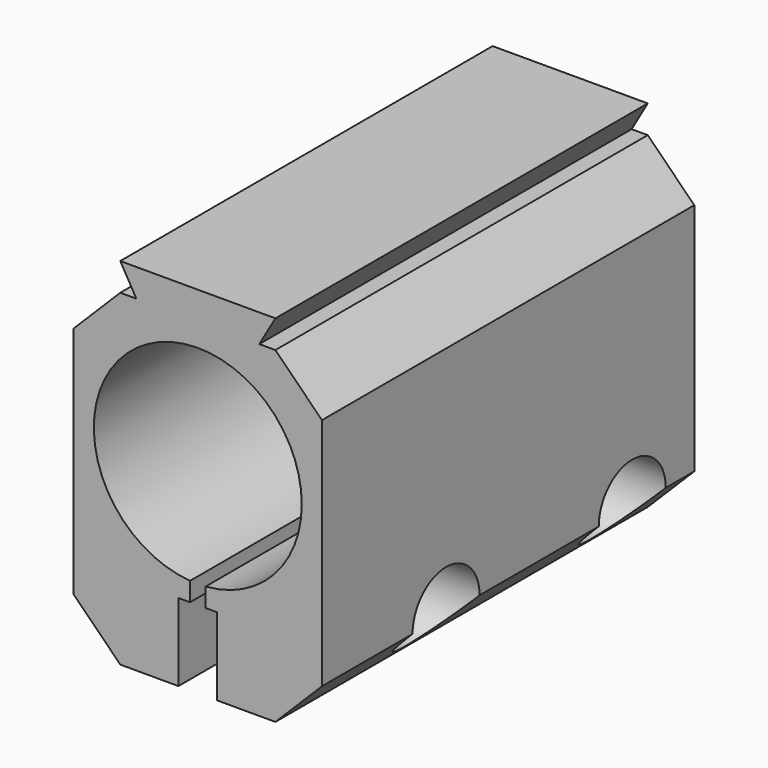
from build123d import *

# Parameters (mm, degrees)
F0_R     = 8.509
F1_DEPTH = 38.1
F3_DEPTH = 6.35
F5_DEPTH = 5.08
F6_DEPTH = 20.321
F8_DEPTH = 8.897727111


# Not quite as in the source:
# - a feature names something its author has since deleted; it is built from what else it names


with BuildPart() as f1:
    # F0 (on Front) → F1 (new body)
    with BuildSketch(Plane.XZ):
        Polygon((5.0301772846, 10.414), (-5.0301772846, 10.414), (-6.35, 10.414), (-10.16, 6.604), (-10.16, -12.5681449387), (-6.3451449387, -16.383), (6.35, -16.383), (10.16, -12.573), (10.16, 6.604), (6.35, 10.414), align=None)
        Circle(F0_R, mode=Mode.SUBTRACT)
        Polygon((6.35, 12.7), (-6.35, 12.7), (-5.0301772846, 10.414), (5.0301772846, 10.414), align=None)
    extrude(amount=F1_DEPTH)

    # F2 (on face) → F3 (cut)
    with BuildSketch(Plane(origin=(0, 0, -16.383), x_dir=(1, 0, 0), z_dir=(0, 0, -1))):
        with BuildLine():
            Line((1.5875, 38.1), (-1.5875, 38.1))
            Line((-1.5875, 38.1), (-1.5875, 22.86))
            ThreePointArc((-1.5875, 22.86), (0, 21.2725), (1.5875, 22.86))
            Line((1.5875, 22.86), (1.5875, 38.1))
        make_face()
    extrude(amount=-F3_DEPTH, mode=Mode.SUBTRACT)

    # F4 (on face) → F5 (cut)
    with BuildSketch(Plane.YZ.offset(10.16)):
        with BuildLine():
            ThreePointArc((-28.829, -12.573), (-25.4, -16.002), (-21.971, -12.573))
            Line((-21.971, -12.573), (-23.495, -12.573))
            ThreePointArc((-23.495, -12.573), (-25.4, -14.478), (-27.305, -12.573))
            Line((-27.305, -12.573), (-28.829, -12.573))
        make_face()
        with BuildLine():
            ThreePointArc((-2.921, -12.573), (-6.35, -9.144), (-9.779, -12.573))
            Line((-9.779, -12.573), (-8.255, -12.573))
            ThreePointArc((-8.255, -12.573), (-6.35, -10.668), (-4.445, -12.573))
            Line((-4.445, -12.573), (-2.921, -12.573))
        make_face()
        with BuildLine():
            Line((-8.255, -12.573), (-9.779, -12.573))
            ThreePointArc((-9.779, -12.573), (-6.35, -16.002), (-2.921, -12.573))
            Line((-2.921, -12.573), (-4.445, -12.573))
            ThreePointArc((-4.445, -12.573), (-6.35, -14.478), (-8.255, -12.573))
        make_face()
        with BuildLine():
            Line((-23.495, -12.573), (-21.971, -12.573))
            ThreePointArc((-21.971, -12.573), (-25.4, -9.144), (-28.829, -12.573))
            Line((-28.829, -12.573), (-27.305, -12.573))
            ThreePointArc((-27.305, -12.573), (-25.4, -10.668), (-23.495, -12.573))
        make_face()
    extrude(amount=-F5_DEPTH, mode=Mode.SUBTRACT)

    # F6 (cut, through all): faces of the model
    f6_faces = [f1.faces().sort_by_distance(p)[0] for p in [
        (10.16, -25.4, -11.7644928891),
        (9.3514928891, -25.4, -13.3815071109),
        (10.16, -6.35, -11.7644928891),
        (9.3514928891, -6.35, -13.3815071109),
    ]]
    extrude(f6_faces, amount=-F6_DEPTH, dir=(1, 0, 0), mode=Mode.SUBTRACT)

    # F7 (on face) → F8 (cut, up to face)
    with BuildSketch(Plane(origin=(0, 0, -16.383), x_dir=(1, 0, 0), z_dir=(0, 0, -1))):
        with BuildLine():
            Line((-0.635, 0), (0.635, 0))
            Line((0.635, 0), (0.635, 21.4050322169))
            ThreePointArc((0.635, 21.4050322169), (0, 21.2725), (-0.635, 21.4050322169))
            Line((-0.635, 21.4050322169), (-0.635, 0))
        make_face()
        with BuildLine():
            ThreePointArc((-0.635, 21.4050322169), (0, 21.2725), (0.635, 21.4050322169))
            Line((0.635, 21.4050322169), (0.635, 38.1))
            Line((0.635, 38.1), (-0.635, 38.1))
            Line((-0.635, 38.1), (-0.635, 21.4050322169))
        make_face()
    extrude(amount=-F8_DEPTH, mode=Mode.SUBTRACT)


solid = f1.part
